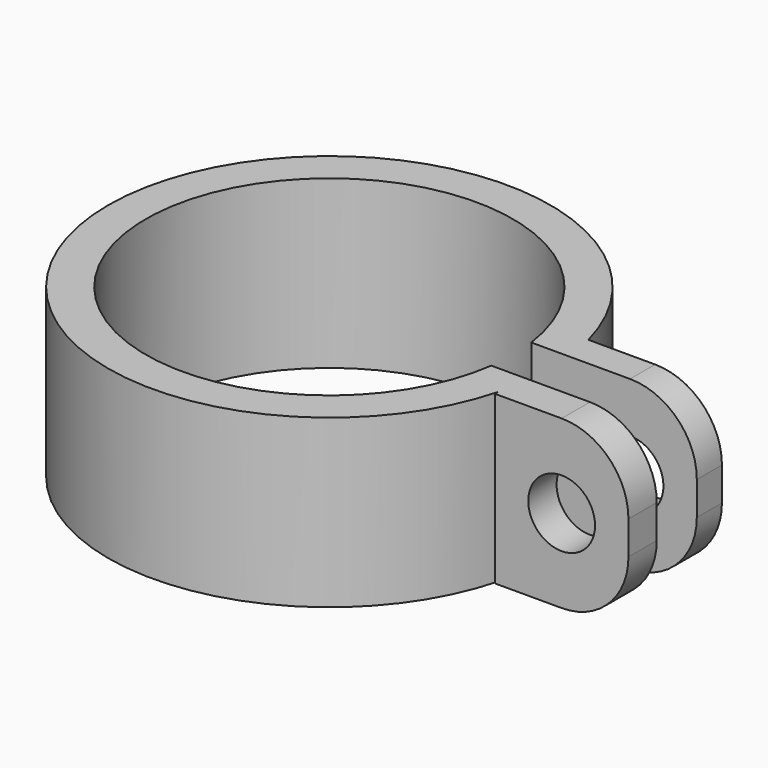
from build123d import *

# Parameters (mm, degrees)
F0_R     = 11
F1_DEPTH = 10
F2_W     = 26.7762894586
F2_H     = 3
F3_DEPTH = 11.5
F4_R     = 2
F5_DEPTH = 25
F6_R     = 4


# Not quite as in the source:
# - a feature names something its author has since deleted; it is built from what else it names


with BuildPart() as f1:
    # F0 (on Top) → F1 (new body)
    with BuildSketch(Plane.XY):
        with BuildLine():
            Line((20.8116516682, 3.3799528892), (12.8116516682, 3.3799528892))
            ThreePointArc((12.8116516682, 3.3799528892), (-13.25, 0), (12.8116516682, -3.3799528892))
            Line((12.8116516682, -3.3799528892), (12.8116516682, -3.6200471108))
            Line((12.8116516682, -3.6200471108), (20.8116516682, -3.6200471108))
            Line((20.8116516682, -3.6200471108), (20.8116516682, 3.3799528892))
        make_face()
        Circle(F0_R, mode=Mode.SUBTRACT)
    extrude(amount=F1_DEPTH)

    # F2 (on Top) → F3 (cut, symmetric)
    with BuildSketch(Plane.XY):
        with Locations((19.2577867381, 0)):
            Rectangle(F2_W, F2_H)
    extrude(amount=F3_DEPTH, both=True, mode=Mode.SUBTRACT)

    # F4 (on face) → F5 (cut)
    with BuildSketch(Plane.XZ.offset(3.6200471108)):
        with Locations((16.8116516682, 5)):
            Circle(F4_R)
    extrude(amount=-F5_DEPTH, mode=Mode.SUBTRACT)

    # F6
    f6_edges = [f1.edges().sort_by_distance(p)[0] for p in [
        (20.811652, -2.560024, 10),
        (20.811652, 2.439976, 10),
        (20.811652, 2.439976, 0),
        (20.811652, -2.560024, 0),
    ]]
    fillet(f6_edges, radius=F6_R)


solid = f1.part
